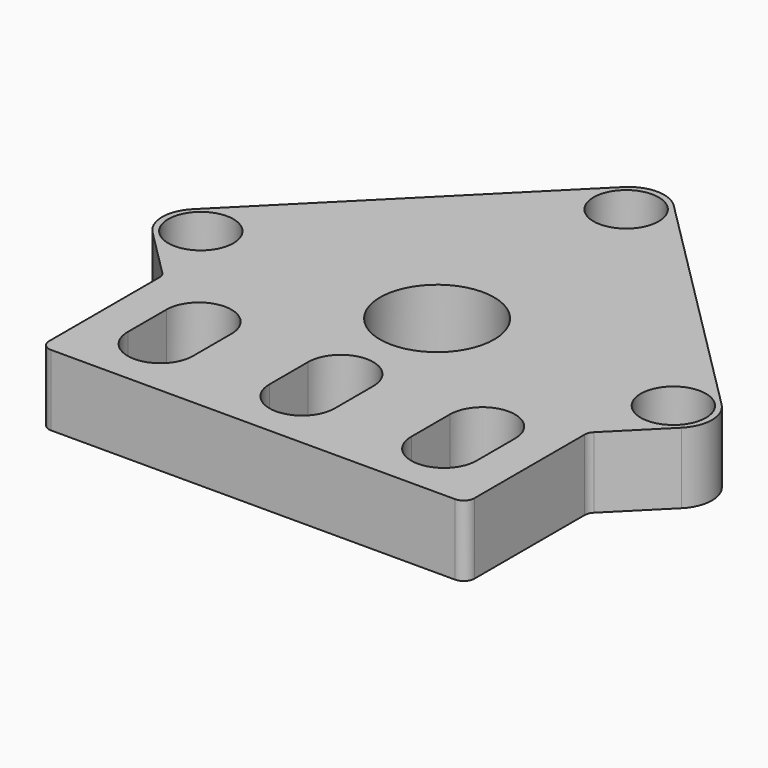
from build123d import *

# Parameters (mm, degrees)
F0_R     = 4.6
F0_R_2   = 8.05
F1_DEPTH = 10
F0_R_3   = 2.5
F2_DEPTH = 3


# Not quite as in the source:
# - ends of sketch curves that miss each other by under 0.0002 mm in the source are joined


with BuildPart() as f1:
    # F0 (on Top) → F1 (new body)
    with BuildSketch(Plane.XY):
        with BuildLine():
            ThreePointArc((-30, -34.104246), (-29.5606601718, -35.1649061718), (-28.5, -35.604246))
            Line((-28.5, -35.604246), (28.5, -35.604246))
            ThreePointArc((28.5, -35.604246), (29.5606601718, -35.1649061718), (30, -34.104246))
            Line((30, -34.104246), (30, -14.645125))
            ThreePointArc((30, -14.645125), (30.1141807012, -14.0710998515), (30.4393398282, -13.5844648282))
            Line((30.4393398282, -13.5844648282), (37.314025, -6.70978))
            ThreePointArc((37.314025, -6.70978), (38.778491, -3.174246), (37.3140249059, 0.3612879059))
            Line((37.3140249059, 0.3612879059), (3.535534, 34.139779))
            ThreePointArc((3.535534, 34.139779), (0, 35.604245), (-3.5355339059, 34.1397789059))
            Line((-3.5355339059, 34.1397789059), (-37.314025, 0.361288))
            ThreePointArc((-37.314025, 0.361288), (-38.778491, -3.174246), (-37.3140249059, -6.7097799059))
            Line((-37.3140249059, -6.7097799059), (-30.43934, -13.584465))
            ThreePointArc((-30.43934, -13.584465), (-30.1141807012, -14.0710998515), (-30, -14.645125))
            Line((-30, -14.645125), (-30, -34.104246))
        make_face()
        with BuildLine():
            ThreePointArc((-24.6, -20.174246), (-20, -15.574246), (-15.4, -20.174246))
            Line((-15.4, -20.174246), (-15.4, -26.974246))
            ThreePointArc((-15.4, -26.974246), (-20, -31.574246), (-24.6, -26.974246))
            Line((-24.6, -26.974246), (-24.6, -20.174246))
        make_face(mode=Mode.SUBTRACT)
        with Locations((-33.333, -3.174246)):
            Circle(F0_R, mode=Mode.SUBTRACT)
        with BuildLine():
            ThreePointArc((4.6, -26.974246), (0, -31.574246), (-4.6, -26.974246))
            Line((-4.6, -26.974246), (-4.6, -20.174246))
            ThreePointArc((-4.6, -20.174246), (0, -15.574246), (4.6, -20.174246))
            Line((4.6, -20.174246), (4.6, -26.974246))
        make_face(mode=Mode.SUBTRACT)
        with BuildLine():
            ThreePointArc((24.6, -26.974246), (20, -31.574246), (15.4, -26.974246))
            Line((15.4, -26.974246), (15.4, -20.174246))
            ThreePointArc((15.4, -20.174246), (20, -15.574246), (24.6, -20.174246))
            Line((24.6, -20.174246), (24.6, -26.974246))
        make_face(mode=Mode.SUBTRACT)
        with Locations((0, -3.174246)):
            Circle(F0_R_2, mode=Mode.SUBTRACT)
        with Locations((33.333, -3.174246)):
            Circle(F0_R, mode=Mode.SUBTRACT)
        with Locations((0, 30.158782)):
            Circle(F0_R, mode=Mode.SUBTRACT)
    extrude(amount=F1_DEPTH)

    # F0 (on Top) → F2 (join)
    with BuildSketch(Plane.XY):
        with Locations((-33.333, -3.174246)):
            Circle(F0_R)
        with Locations((-33.333, -3.174246)):
            Circle(F0_R_3, mode=Mode.SUBTRACT)
        with BuildLine():
            Line((-15.4, -26.974246), (-15.4, -20.174246))
            ThreePointArc((-15.4, -20.174246), (-20, -15.574246), (-24.6, -20.174246))
            Line((-24.6, -20.174246), (-24.6, -26.974246))
            ThreePointArc((-24.6, -26.974246), (-20, -31.574246), (-15.4, -26.974246))
        make_face()
        with BuildLine():
            ThreePointArc((-17.5, -26.974246), (-20, -29.474246), (-22.5, -26.974246))
            Line((-22.5, -26.974246), (-22.5, -20.174246))
            ThreePointArc((-22.5, -20.174246), (-20, -17.674246), (-17.5, -20.174246))
            Line((-17.5, -20.174246), (-17.5, -26.974246))
        make_face(mode=Mode.SUBTRACT)
        with BuildLine():
            Line((-4.6, -20.174246), (-4.6, -26.974246))
            ThreePointArc((-4.6, -26.974246), (0, -31.574246), (4.6, -26.974246))
            Line((4.6, -26.974246), (4.6, -20.174246))
            ThreePointArc((4.6, -20.174246), (0, -15.574246), (-4.6, -20.174246))
        make_face()
        with BuildLine():
            ThreePointArc((2.5, -26.974246), (0, -29.474246), (-2.5, -26.974246))
            Line((-2.5, -26.974246), (-2.5, -20.174246))
            ThreePointArc((-2.5, -20.174246), (0, -17.674246), (2.5, -20.174246))
            Line((2.5, -20.174246), (2.5, -26.974246))
        make_face(mode=Mode.SUBTRACT)
        with BuildLine():
            Line((15.4, -20.174246), (15.4, -26.974246))
            ThreePointArc((15.4, -26.974246), (20, -31.574246), (24.6, -26.974246))
            Line((24.6, -26.974246), (24.6, -20.174246))
            ThreePointArc((24.6, -20.174246), (20, -15.574246), (15.4, -20.174246))
        make_face()
        with BuildLine():
            ThreePointArc((22.5, -26.974246), (20, -29.474246), (17.5, -26.974246))
            Line((17.5, -26.974246), (17.5, -20.174246))
            ThreePointArc((17.5, -20.174246), (20, -17.674246), (22.5, -20.174246))
            Line((22.5, -20.174246), (22.5, -26.974246))
        make_face(mode=Mode.SUBTRACT)
        with Locations((33.333, -3.174246)):
            Circle(F0_R)
        with Locations((33.333, -3.174246)):
            Circle(F0_R_3, mode=Mode.SUBTRACT)
        with Locations((0, 30.158782)):
            Circle(F0_R)
        with Locations((0, 30.158782)):
            Circle(F0_R_3, mode=Mode.SUBTRACT)
    extrude(amount=F2_DEPTH)


solid = f1.part
